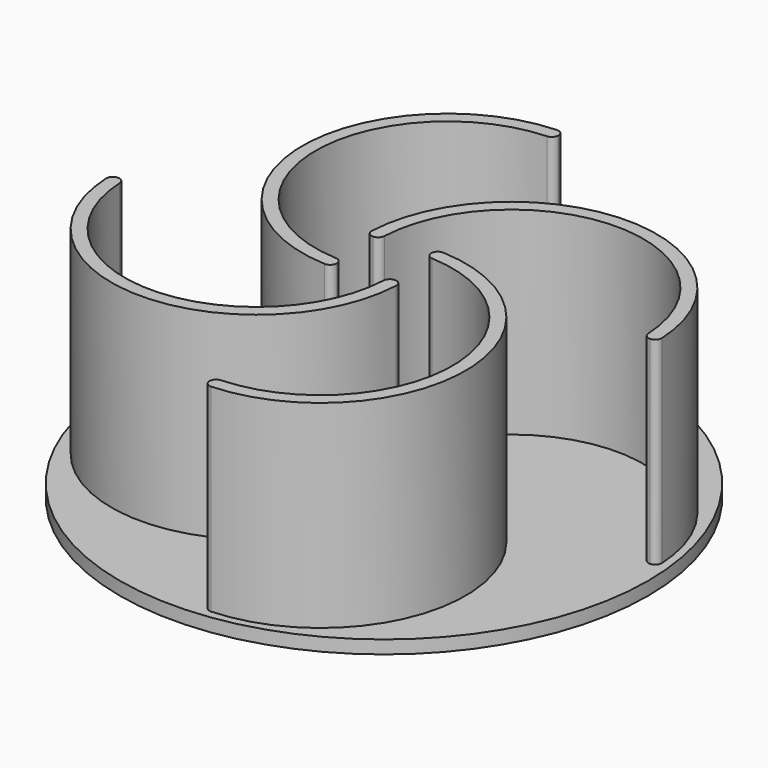
from build123d import *

# Parameters (mm, degrees)
F1_DEPTH = 30
F2_R     = 0.99999
F2_2_R   = 0.99999
F2_3_R   = 0.99999
F2_4_R   = 0.99999
F3_R     = 40
F4_DEPTH = 2
F5_DEPTH = 25


# Not quite as in the source:
# - a fillet or chamfer is up to 0.001 mm smaller than in the source, because OpenCascade refuses the exact size


with BuildPart() as f1:
    # F0 (on Top) → F1 (new body)
    with BuildSketch(Plane.XY):
        with BuildLine():
            Line((-5.5355339059, 3.5355339059), (-3.5355339059, 3.5355339059))
            ThreePointArc((-3.5355339059, 3.5355339059), (16.4644660941, 23.5355339059), (36.4644660941, 3.5355339059))
            Line((36.4644660941, 3.5355339059), (38.4644660941, 3.5355339059))
            ThreePointArc((38.4644660941, 3.5355339059), (16.4644660941, 25.5355339059), (-5.5355339059, 3.5355339059))
        make_face()
    extrude(amount=F1_DEPTH)

    # F2 (radius 1 in the source; OpenCascade refuses exactly that, so slightly less here)
    f2_edges = [f1.edges().sort_by_distance(p)[0] for p in [
        (-3.535534, 3.535534, 15),
        (-5.535534, 3.535534, 15),
        (38.464466, 3.535534, 15),
        (36.464466, 3.535534, 15),
    ]]
    fillet(f2_edges, radius=F2_R)



with BuildPart() as f1b:
    # F0 (on Top) → F1, piece 2 (new body)
    with BuildSketch(Plane.XY):
        with BuildLine():
            Line((3.5355339059, 5.5355339059), (3.5355339059, 3.5355339059))
            ThreePointArc((3.5355339059, 3.5355339059), (23.5355339059, -16.4644660941), (3.5355339059, -36.4644660941))
            Line((3.5355339059, -36.4644660941), (3.5355339059, -38.4644660941))
            ThreePointArc((3.5355339059, -38.4644660941), (25.5355339059, -16.4644660941), (3.5355339059, 5.5355339059))
        make_face()
    extrude(amount=F1_DEPTH)

    # F2#2 (radius 1 in the source; OpenCascade refuses exactly that, so slightly less here)
    f2_2_edges = [f1b.edges().sort_by_distance(p)[0] for p in [
        (3.535534, 3.535534, 15),
        (3.535534, 5.535534, 15),
        (3.535534, -38.464466, 15),
        (3.535534, -36.464466, 15),
    ]]
    fillet(f2_2_edges, radius=F2_2_R)


with BuildPart() as f1c:
    # F0 (on Top) → F1, piece 3 (new body)
    with BuildSketch(Plane.XY):
        with BuildLine():
            Line((-3.5355339059, -5.5355339059), (-3.5355339059, -3.5355339059))
            ThreePointArc((-3.5355339059, -3.5355339059), (-23.5355339059, 16.4644660941), (-3.5355339059, 36.4644660941))
            Line((-3.5355339059, 36.4644660941), (-3.5355339059, 38.4644660941))
            ThreePointArc((-3.5355339059, 38.4644660941), (-25.5355339059, 16.4644660941), (-3.5355339059, -5.5355339059))
        make_face()
    extrude(amount=F1_DEPTH)

    # F2#4 (radius 1 in the source; OpenCascade refuses exactly that, so slightly less here)
    f2_4_edges = [f1c.edges().sort_by_distance(p)[0] for p in [
        (-3.535534, -3.535534, 15),
        (-3.535534, -5.535534, 15),
        (-3.535534, 38.464466, 15),
        (-3.535534, 36.464466, 15),
    ]]
    fillet(f2_4_edges, radius=F2_4_R)


with BuildPart() as f1d:
    # F0 (on Top) → F1, piece 4 (new body)
    with BuildSketch(Plane.XY):
        with BuildLine():
            Line((5.5355339059, -3.5355339059), (3.5355339059, -3.5355339059))
            ThreePointArc((3.5355339059, -3.5355339059), (-16.4644660941, -23.5355339059), (-36.4644660941, -3.5355339059))
            Line((-36.4644660941, -3.5355339059), (-38.4644660941, -3.5355339059))
            ThreePointArc((-38.4644660941, -3.5355339059), (-16.4644660941, -25.5355339059), (5.5355339059, -3.5355339059))
        make_face()
    extrude(amount=F1_DEPTH)

    # F2#3 (radius 1 in the source; OpenCascade refuses exactly that, so slightly less here)
    f2_3_edges = [f1d.edges().sort_by_distance(p)[0] for p in [
        (3.535534, -3.535534, 15),
        (5.535534, -3.535534, 15),
        (-38.464466, -3.535534, 15),
        (-36.464466, -3.535534, 15),
    ]]
    fillet(f2_3_edges, radius=F2_3_R)


with BuildPart() as f1_1:
    add(f1.part)

    add(f1b.part)  # F4 merges F1b

    add(f1c.part)  # F4 merges F1c

    add(f1d.part)  # F4 merges F1d
    # F3 (on Top) → F4 (join)
    with BuildSketch(Plane.XY):
        Circle(F3_R)
    extrude(amount=-F4_DEPTH)

    # F0 (on Top) → F5 (cut)
    with BuildSketch(Plane.XY):
        Polygon((-3.5355339059, -3.5355339059), (3.5355339059, -3.5355339059), (0, 0), align=None)
        with BuildLine():
            ThreePointArc((-3.5355339059, -3.5355339059), (0, -5), (3.5355339059, -3.5355339059))
            Line((3.5355339059, -3.5355339059), (-3.5355339059, -3.5355339059))
        make_face()
        Polygon((0, 0), (-3.5355339059, 3.5355339059), (-3.5355339059, -3.5355339059), align=None)
        with BuildLine():
            Line((-3.5355339059, -3.5355339059), (-3.5355339059, 3.5355339059))
            ThreePointArc((-3.5355339059, 3.5355339059), (-5, 0), (-3.5355339059, -3.5355339059))
        make_face()
        Polygon((0, 0), (3.5355339059, 3.5355339059), (-3.5355339059, 3.5355339059), align=None)
        with BuildLine():
            Line((-3.5355339059, 3.5355339059), (3.5355339059, 3.5355339059))
            ThreePointArc((3.5355339059, 3.5355339059), (0, 5), (-3.5355339059, 3.5355339059))
        make_face()
        Polygon((3.5355339059, -3.5355339059), (3.5355339059, 3.5355339059), (0, 0), align=None)
        with BuildLine():
            ThreePointArc((3.5355339059, -3.5355339059), (4.6193976626, -1.9134171618), (5, 0))
            ThreePointArc((5, 0), (4.6193976626, 1.9134171618), (3.5355339059, 3.5355339059))
            Line((3.5355339059, 3.5355339059), (3.5355339059, -3.5355339059))
        make_face()
    extrude(amount=-F5_DEPTH, mode=Mode.SUBTRACT)


solid = f1_1.part
